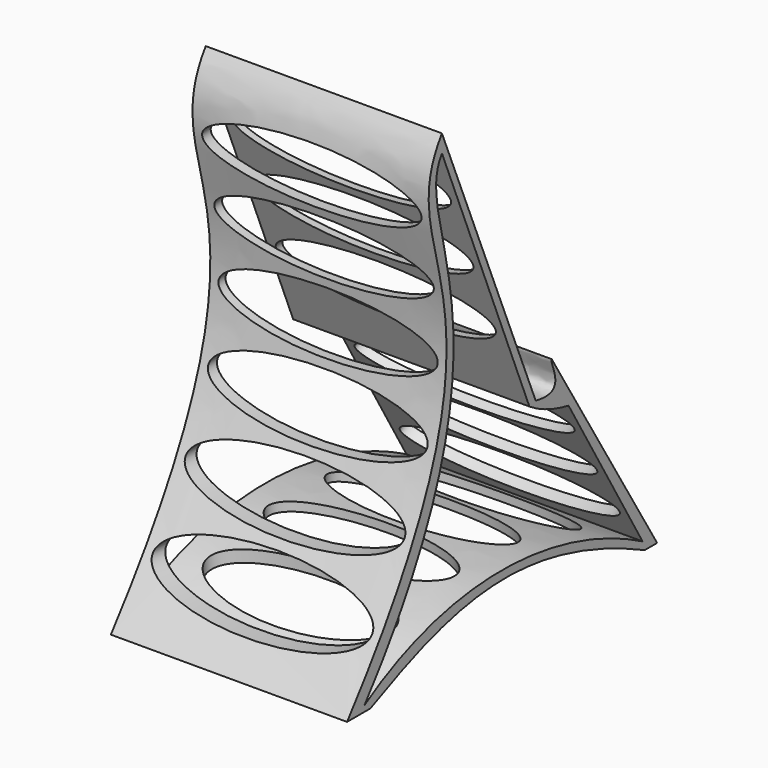
from build123d import *

# Parameters (mm, degrees)
F1_DEPTH  = 70
F3_REACH  = 140.8427948945
F5_REACH  = 198.6043545962
F8_REACH  = 187.2157962538
F9_REACH  = 187.2157962538
F12_REACH = 200.5256779964


with BuildPart() as f1:
    # F0 (on Right) → F1 (new body)
    with BuildSketch(Plane.YZ):
        with BuildLine():
            add(Edge.make_bspline(
                [(-65.0536715984, 0), (5.2683912218, 89.8734778166), (-50.6073869765, 110.0246235728), (-29.9188829958, 139.2738819122)],
                knots=[0, 0, 0, 0, 143.6372777278, 143.6372777278, 143.6372777278, 143.6372777278], degree=3))
            Line((-65.0536715984, 0), (-56.4117916499, 0))
            add(Edge.make_bspline(
                [(-56.4117916499, 0), (-27.936052531, 13.126176782), (-1.7122571589, 22.8152908385), (45.2086254954, 0)],
                knots=[0, 0, 0, 0, 101.6204171453, 101.6204171453, 101.6204171453, 101.6204171453], degree=3))
            Line((45.2086254954, 0), (49.8031899333, 0))
            add(Edge.make_bspline(
                [(49.8031899333, 0), (36.7837014298, 21.2773953875), (23.7642129262, 42.554790775), (10.7447244227, 63.8321861625)],
                knots=[0, 0, 0, 0, 74.8338941812, 74.8338941812, 74.8338941812, 74.8338941812], degree=3))
            add(Edge.make_bspline(
                [(4.8285723044, 55.386091928), (17.0853175535, 52.8970839186), (9.9300900474, 62.5007674098), (10.7447244227, 63.8321861625)],
                knots=[0, 0, 0, 0, 10.3120009554, 10.3120009554, 10.3120009554, 10.3120009554], degree=3))
            Line((4.8285723044, 55.386091928), (-29.9188829958, 139.2738819122))
        make_face()
        with BuildLine():
            add(Edge.make_bspline(
                [(-58.5831403732, 1.7520016991), (-26.5599957202, 21.9477838837), (12.6107810065, 19.9717469513), (44.4163493812, 2.5945331436)],
                knots=[0, 0, 0, 0, 103.0029356325, 103.0029356325, 103.0029356325, 103.0029356325], degree=3))
            add(Edge.make_bspline(
                [(-58.5831403732, 1.7520016991), (1.96994422, 79.0443941951), (-41.790433228, 117.2437295318), (-29.9037508667, 134.0290158987)],
                knots=[0, 0, 0, 0, 135.3503449129, 135.3503449129, 135.3503449129, 135.3503449129], degree=3))
            Line((-29.9037508667, 134.0290158987), (2.4867416879, 54.8259804102))
            add(Edge.make_bspline(
                [(2.4867416879, 54.8259804102), (6.9520277902, 51.7374575138), (13.1526212381, 49.8405049891), (16.9847030193, 49.1881705821)],
                knots=[0, 0, 0, 0, 15.5555707843, 15.5555707843, 15.5555707843, 15.5555707843], degree=3))
            Line((16.9847030193, 49.1881705821), (44.4163493812, 2.5945331436))
        make_face(mode=Mode.SUBTRACT)
    extrude(amount=F1_DEPTH)

    f3_end = f1.faces().sort_by_distance((35, 30.273957178, 31.9160930812))[0]
    # F2 (on face) → F3 (cut, up to a face of the model that its end follows)
    with BuildSketch(Plane(origin=(0, 34.1179734072, 20.086694934), x_dir=(1, 0, 0), z_dir=(0, -0.8617432082, -0.5073446986))):
        with BuildLine():
            add(Edge.make_bspline(
                [(67.5, 23.4277807176), (67.5, 36.9762650043), (18.75, 30.202022861), (-30, 23.4277807176), (18.75, 16.6535385743), (67.5, 9.8792964309), (67.5, 23.4277807176)],
                knots=[0, 0, 0, 2.0943951024, 2.0943951024, 4.1887902048, 4.1887902048, 6.2831853072, 6.2831853072, 6.2831853072], degree=2, weights=[1, 0.5, 1, 0.5, 1, 0.5, 1]))
        make_face()
        with BuildLine():
            add(Edge.make_bspline(
                [(67.5, 6.9277807176), (67.5, 20.4762650043), (18.75, 13.702022861), (-30, 6.9277807176), (18.75, 0.1535385743), (67.5, -6.6207035691), (67.5, 6.9277807176)],
                knots=[0, 0, 0, 2.0943951024, 2.0943951024, 4.1887902048, 4.1887902048, 6.2831853072, 6.2831853072, 6.2831853072], degree=2, weights=[1, 0.5, 1, 0.5, 1, 0.5, 1]))
        make_face()
        with BuildLine():
            add(Edge.make_bspline(
                [(67.5, -9.5722192824), (67.5, 3.9762650043), (18.75, -2.797977139), (-30, -9.5722192824), (18.75, -16.3464614257), (67.5, -23.1207035691), (67.5, -9.5722192824)],
                knots=[0, 0, 0, 2.0943951024, 2.0943951024, 4.1887902048, 4.1887902048, 6.2831853072, 6.2831853072, 6.2831853072], degree=2, weights=[1, 0.5, 1, 0.5, 1, 0.5, 1]))
        make_face()
    f3_long = extrude(amount=-F3_REACH, mode=Mode.PRIVATE)
    add(split(f3_long, bisect_by=f3_end, keep=Keep.BOTTOM, mode=Mode.PRIVATE), mode=Mode.SUBTRACT)

    f5_end = f1.faces().sort_by_distance((35, -7.0018043916, 16.2631409185))[0]
    # F4 (on Top) → F5 (cut, up to a face of the model that its end follows)
    with BuildSketch(Plane.XY):
        with BuildLine():
            add(Edge.make_bspline(
                [(62.8528258204, -38.5428890586), (62.8528258204, -20.8609774983), (21.0735870898, -29.7019332784), (-20.7056516409, -38.5428890586), (21.0735870898, -47.3838448388), (62.8528258204, -56.2248006189), (62.8528258204, -38.5428890586)],
                knots=[0, 0, 0, 2.0943951024, 2.0943951024, 4.1887902048, 4.1887902048, 6.2831853072, 6.2831853072, 6.2831853072], degree=2, weights=[1, 0.5, 1, 0.5, 1, 0.5, 1]))
        make_face()
        with BuildLine():
            add(Edge.make_bspline(
                [(62.8528258204, -15.9428890586), (62.8528258204, 1.7390225017), (21.0735870898, -7.1019332784), (-20.7056516409, -15.9428890586), (21.0735870898, -24.7838448388), (62.8528258204, -33.6248006189), (62.8528258204, -15.9428890586)],
                knots=[0, 0, 0, 2.0943951024, 2.0943951024, 4.1887902048, 4.1887902048, 6.2831853072, 6.2831853072, 6.2831853072], degree=2, weights=[1, 0.5, 1, 0.5, 1, 0.5, 1]))
        make_face()
        with BuildLine():
            add(Edge.make_bspline(
                [(62.8528258204, 6.6571109414), (62.8528258204, 24.3390225017), (21.0735870898, 15.4980667216), (-20.7056516409, 6.6571109414), (21.0735870898, -2.1838448388), (62.8528258204, -11.0248006189), (62.8528258204, 6.6571109414)],
                knots=[0, 0, 0, 2.0943951024, 2.0943951024, 4.1887902048, 4.1887902048, 6.2831853072, 6.2831853072, 6.2831853072], degree=2, weights=[1, 0.5, 1, 0.5, 1, 0.5, 1]))
        make_face()
        with BuildLine():
            add(Edge.make_bspline(
                [(62.8528258204, 29.2571109414), (62.8528258204, 46.9390225017), (21.0735870898, 38.0980667216), (-20.7056516409, 29.2571109414), (21.0735870898, 20.4161551612), (62.8528258204, 11.5751993811), (62.8528258204, 29.2571109414)],
                knots=[0, 0, 0, 2.0943951024, 2.0943951024, 4.1887902048, 4.1887902048, 6.2831853072, 6.2831853072, 6.2831853072], degree=2, weights=[1, 0.5, 1, 0.5, 1, 0.5, 1]))
        make_face()
    f5_long = extrude(amount=F5_REACH, mode=Mode.PRIVATE)
    add(split(f5_long, bisect_by=f5_end, keep=Keep.BOTTOM, mode=Mode.PRIVATE), mode=Mode.SUBTRACT)

    f8_end = f1.faces().sort_by_distance((35, -25.993544783, 90.5806735973))[0]
    # F7 (on offset) → F8 (cut, up to a face of the model that its end follows)
    with BuildSketch(Plane.XZ.offset(70)):
        with BuildLine():
            add(Edge.make_bspline(
                [(67.5, 57.6202747583), (67.5, 73.0958511632), (18.75, 65.3580629608), (-30, 57.6202747583), (18.75, 49.8824865559), (67.5, 42.1446983534), (67.5, 57.6202747583)],
                knots=[0, 0, 0, 2.0943951024, 2.0943951024, 4.1887902048, 4.1887902048, 6.2831853072, 6.2831853072, 6.2831853072], degree=2, weights=[1, 0.5, 1, 0.5, 1, 0.5, 1]))
        make_face()
        with BuildLine():
            add(Edge.make_bspline(
                [(67.5, 37.3202747583), (67.5, 52.7958511632), (18.75, 45.0580629608), (-30, 37.3202747583), (18.75, 29.5824865559), (67.5, 21.8446983534), (67.5, 37.3202747583)],
                knots=[0, 0, 0, 2.0943951024, 2.0943951024, 4.1887902048, 4.1887902048, 6.2831853072, 6.2831853072, 6.2831853072], degree=2, weights=[1, 0.5, 1, 0.5, 1, 0.5, 1]))
        make_face()
        with BuildLine():
            add(Edge.make_bspline(
                [(67.5, 17.0202747583), (67.5, 32.4958511632), (18.75, 24.7580629608), (-30, 17.0202747583), (18.75, 9.2824865559), (67.5, 1.5446983534), (67.5, 17.0202747583)],
                knots=[0, 0, 0, 2.0943951024, 2.0943951024, 4.1887902048, 4.1887902048, 6.2831853072, 6.2831853072, 6.2831853072], degree=2, weights=[1, 0.5, 1, 0.5, 1, 0.5, 1]))
        make_face()
    f8_long = extrude(amount=-F8_REACH, mode=Mode.PRIVATE)
    add(split(f8_long, bisect_by=f8_end, keep=Keep.BOTTOM, mode=Mode.PRIVATE), mode=Mode.SUBTRACT)

    f9_end = f1.faces().sort_by_distance((35, -12.5451553457, 97.3299869201))[0]
    # F7 (on offset) → F9 (cut, up to a face of the model that its end follows)
    with BuildSketch(Plane.XZ.offset(70)):
        with BuildLine():
            add(Edge.make_bspline(
                [(67.5, 118.5202747583), (67.5, 133.9958511632), (18.75, 126.2580629608), (-30, 118.5202747583), (18.75, 110.7824865559), (67.5, 103.0446983534), (67.5, 118.5202747583)],
                knots=[0, 0, 0, 2.0943951024, 2.0943951024, 4.1887902048, 4.1887902048, 6.2831853072, 6.2831853072, 6.2831853072], degree=2, weights=[1, 0.5, 1, 0.5, 1, 0.5, 1]))
        make_face()
        with BuildLine():
            add(Edge.make_bspline(
                [(67.5, 98.2202747583), (67.5, 113.6958511632), (18.75, 105.9580629608), (-30, 98.2202747583), (18.75, 90.4824865559), (67.5, 82.7446983534), (67.5, 98.2202747583)],
                knots=[0, 0, 0, 2.0943951024, 2.0943951024, 4.1887902048, 4.1887902048, 6.2831853072, 6.2831853072, 6.2831853072], degree=2, weights=[1, 0.5, 1, 0.5, 1, 0.5, 1]))
        make_face()
        with BuildLine():
            add(Edge.make_bspline(
                [(67.5, 77.9202747583), (67.5, 93.3958511632), (18.75, 85.6580629608), (-30, 77.9202747583), (18.75, 70.1824865559), (67.5, 62.4446983534), (67.5, 77.9202747583)],
                knots=[0, 0, 0, 2.0943951024, 2.0943951024, 4.1887902048, 4.1887902048, 6.2831853072, 6.2831853072, 6.2831853072], degree=2, weights=[1, 0.5, 1, 0.5, 1, 0.5, 1]))
        make_face()
    f9_long = extrude(amount=-F9_REACH, mode=Mode.PRIVATE)
    add(split(f9_long, bisect_by=f9_end, keep=Keep.BOTTOM, mode=Mode.PRIVATE), mode=Mode.SUBTRACT)

    f12_end = f1.faces().sort_by_distance((35, 9.973173974, 51.0935048126))[0]
    # F11 (on face) → F12 (cut, up to a face of the model that its end follows)
    with BuildSketch(Plane(origin=(0, -53.6222660217, 129.4556206097), x_dir=(1, 0, 0), z_dir=(0, -0.3826833851, 0.9238795521))):
        with BuildLine():
            add(Edge.make_bspline(
                [(14.718651472, 29.656356364), (14.718651472, 22.7281531337), (45.140674264, 26.1922547488), (75.562697056, 29.656356364), (45.140674264, 33.1204579791), (14.718651472, 36.5845595942), (14.718651472, 29.656356364)],
                knots=[0, 0, 0, 2.0943951024, 2.0943951024, 4.1887902048, 4.1887902048, 6.2831853072, 6.2831853072, 6.2831853072], degree=2, weights=[1, 0.5, 1, 0.5, 1, 0.5, 1]))
        make_face()
    f12_long = extrude(amount=-F12_REACH, mode=Mode.PRIVATE)
    add(split(f12_long, bisect_by=f12_end, keep=Keep.BOTTOM, mode=Mode.PRIVATE), mode=Mode.SUBTRACT)


solid = f1.part
